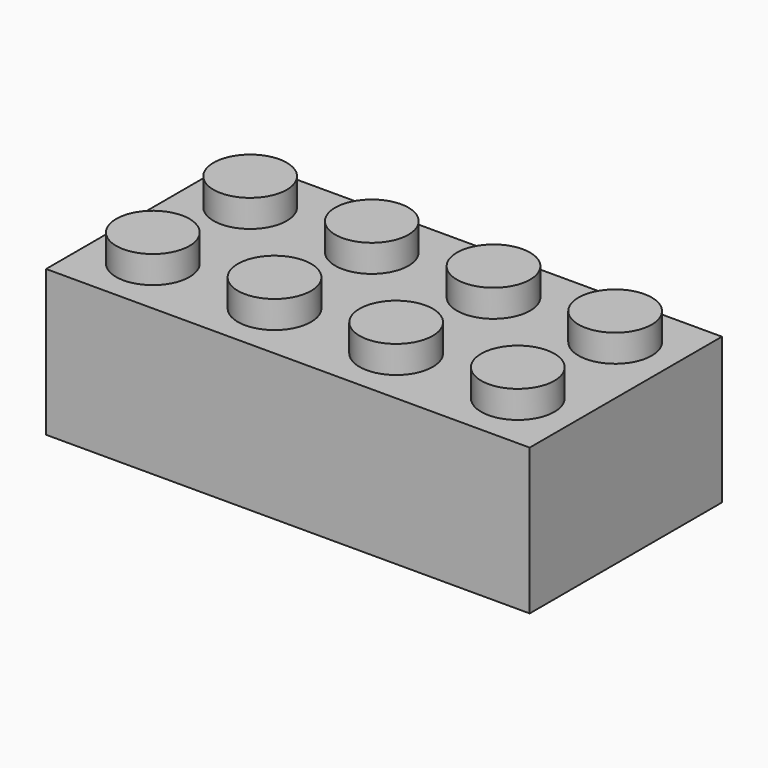
from build123d import *

# Parameters (mm, degrees)
F0_W      = 31.8
F0_H      = 15.8
F1_DEPTH  = 4.8
F2_W      = 29.4
F2_H      = 13.4
F3_DEPTH  = 8.4
F4_R      = 2.409
F5_DEPTH  = 1.8
F6_R      = 1.3
F7_DEPTH  = 1.2
F8_R      = 3.255
F8_R_2    = 2.4
F9_DEPTH  = 8.4
F10_W     = 0.3
F10_H     = 0.6
F11_DEPTH = 8.4
F12_W     = 0.6
F12_H     = 0.3
F13_DEPTH = 8.4
F14_W     = 0.8
F14_H     = 3.4696710694
F15_DEPTH = 6.4


with BuildPart() as f1:
    # F0 (on Top) → F1 (new body, symmetric)
    with BuildSketch(Plane.XY):
        Rectangle(F0_W, F0_H)
    extrude(amount=F1_DEPTH, both=True)

    # F2 (on face) → F3 (cut)
    with BuildSketch(Plane(origin=(0, 0, -4.8), x_dir=(1, 0, 0), z_dir=(0, 0, -1))):
        Rectangle(F2_W, F2_H)
    extrude(amount=-F3_DEPTH, mode=Mode.SUBTRACT)

    # F4 (on face) → F5 (join)
    with BuildSketch(Plane.XY.offset(4.8)):
        with Locations((-12, 4)):
            Circle(F4_R)
        with Locations((-4, 4)):
            Circle(F4_R)
        with Locations((-4, -4)):
            Circle(F4_R)
        with Locations((-12, -4)):
            Circle(F4_R)
        with Locations((4, -4)):
            Circle(F4_R)
        with Locations((12, -4)):
            Circle(F4_R)
        with Locations((4, 4)):
            Circle(F4_R)
        with Locations((12, 4)):
            Circle(F4_R)
    extrude(amount=F5_DEPTH)

    # F6 (on face) → F7 (cut)
    with BuildSketch(Plane(origin=(0, 0, 3.6), x_dir=(1, 0, 0), z_dir=(0, 0, -1))):
        with Locations((-12, 4)):
            Circle(F6_R)
        with Locations((-4, 4)):
            Circle(F6_R)
        with Locations((-4, -4)):
            Circle(F6_R)
        with Locations((-12, -4)):
            Circle(F6_R)
        with Locations((4, -4)):
            Circle(F6_R)
        with Locations((12, -4)):
            Circle(F6_R)
        with Locations((4, 4)):
            Circle(F6_R)
        with Locations((12, 4)):
            Circle(F6_R)
    extrude(amount=-F7_DEPTH, mode=Mode.SUBTRACT)

    # F8 (on face) → F9 (join, through all)
    with BuildSketch(Plane(origin=(0, 0, 3.6), x_dir=(1, 0, 0), z_dir=(0, 0, -1))):
        with Locations((-8, 0)):
            Circle(F8_R)
        with Locations((-8, 0)):
            Circle(F8_R_2, mode=Mode.SUBTRACT)
        Circle(F8_R)
        Circle(F8_R_2, mode=Mode.SUBTRACT)
        with Locations((8, 0)):
            Circle(F8_R)
        with Locations((8, 0)):
            Circle(F8_R_2, mode=Mode.SUBTRACT)
    extrude(amount=F9_DEPTH)

    # F10 (on face) → F11 (join, through all)
    with BuildSketch(Plane(origin=(0, 0, 3.6), x_dir=(1, 0, 0), z_dir=(0, 0, -1))):
        with Locations((-14.55, 4)):
            Rectangle(F10_W, F10_H)
        with Locations((-14.55, -4)):
            Rectangle(F10_W, F10_H)
        with Locations((14.55, 4)):
            Rectangle(F10_W, F10_H)
        with Locations((14.55, -4)):
            Rectangle(F10_W, F10_H)
    extrude(amount=F11_DEPTH)

    # F12 (on face) → F13 (join, through all)
    with BuildSketch(Plane(origin=(0, 0, 3.6), x_dir=(1, 0, 0), z_dir=(0, 0, -1))):
        with Locations((-12, 6.55)):
            Rectangle(F12_W, F12_H)
        with Locations((-12, -6.55)):
            Rectangle(F12_W, F12_H)
        with Locations((-4, 6.55)):
            Rectangle(F12_W, F12_H)
        with Locations((-4, -6.55)):
            Rectangle(F12_W, F12_H)
        with Locations((4, 6.55)):
            Rectangle(F12_W, F12_H)
        with Locations((12, 6.55)):
            Rectangle(F12_W, F12_H)
        with Locations((12, -6.55)):
            Rectangle(F12_W, F12_H)
        with Locations((4, -6.55)):
            Rectangle(F12_W, F12_H)
    extrude(amount=F13_DEPTH)

    # F14 (on face) → F15 (join)
    with BuildSketch(Plane(origin=(0, 0, 3.6), x_dir=(1, 0, 0), z_dir=(0, 0, -1))):
        with Locations((0, 4.9651644653)):
            Rectangle(F14_W, F14_H)
        with Locations((0, -4.9651644653)):
            Rectangle(F14_W, F14_H)
    extrude(amount=F15_DEPTH)


solid = f1.part
